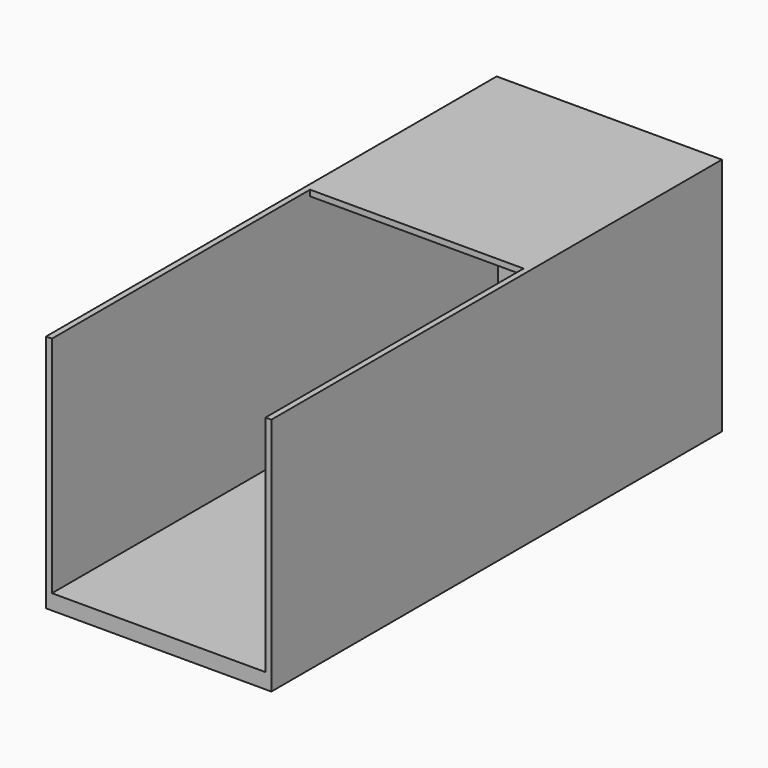
from build123d import *

# Parameters (mm, degrees)
F0_W     = 2438.4
F0_H     = 2590.8
F1_DEPTH = 6096
F2_W     = 2311.4
F2_H     = 2425.7
F3_DEPTH = 6032.5
F4_W     = 2311.4
F4_H     = 63.5
F5_DEPTH = 2540


# Not quite as in the source:
# - a feature names something its author has since deleted; it is built from what else it names


with BuildPart() as f1:
    # F0 (on Front) → F1 (new body)
    with BuildSketch(Plane.XZ):
        with Locations((1219.2, 1295.4)):
            Rectangle(F0_W, F0_H)
    extrude(amount=F1_DEPTH)

    # F2 (on face) → F3 (cut)
    with BuildSketch(Plane.XZ.offset(6096)):
        with Locations((1219.2, 1377.95)):
            Rectangle(F2_W, F2_H)
    extrude(amount=-F3_DEPTH, mode=Mode.SUBTRACT)

    # F4 (on face) → F5 (join)
    with BuildSketch(Plane.XZ.offset(63.5)):
        with Locations((1219.2, 2559.05)):
            Rectangle(F4_W, F4_H)
    extrude(amount=F5_DEPTH)


solid = f1.part
